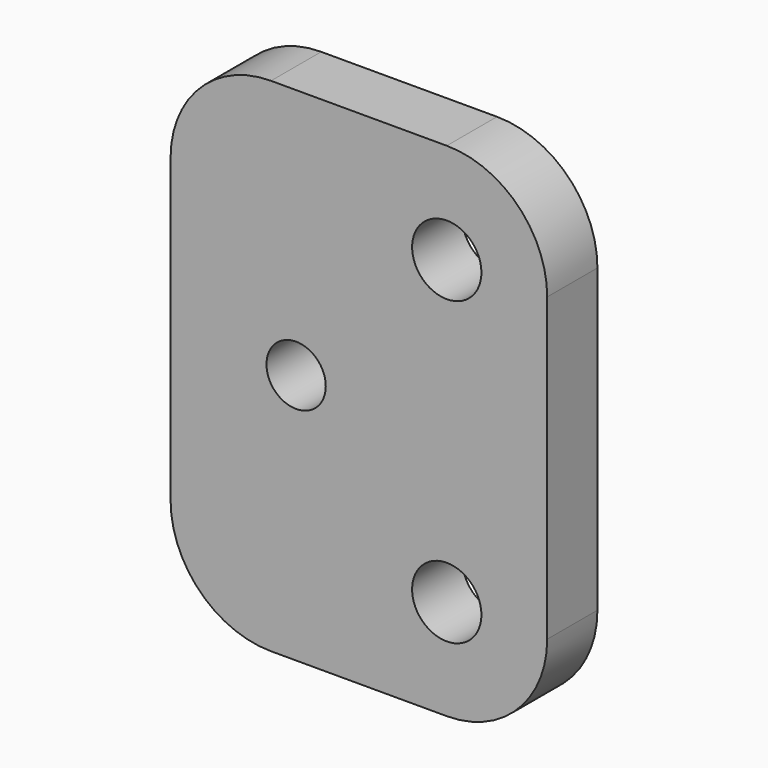
from build123d import *

# Parameters (mm, degrees)
F0_W     = 19.05
F0_H     = 25.4
F0_R     = 1.5
F0_R_2   = 1.7526
F1_DEPTH = 3.175
F2_R     = 5.08


with BuildPart() as f1:
    # F0 (on Front) → F1 (new body)
    with BuildSketch(Plane.XZ):
        with Locations((3.175, 0)):
            Rectangle(F0_W, F0_H)
        Circle(F0_R, mode=Mode.SUBTRACT)
        with Locations((7.62, -7.62)):
            Circle(F0_R_2, mode=Mode.SUBTRACT)
        with Locations((7.62, 7.62)):
            Circle(F0_R_2, mode=Mode.SUBTRACT)
    extrude(amount=F1_DEPTH)

    # F2
    f2_edges = [f1.edges().sort_by_distance(p)[0] for p in [
        (12.7, -1.5875, 12.7),
        (12.7, -1.5875, -12.7),
        (-6.35, -1.5875, 12.7),
        (-6.35, -1.5875, -12.7),
    ]]
    fillet(f2_edges, radius=F2_R)


solid = f1.part
